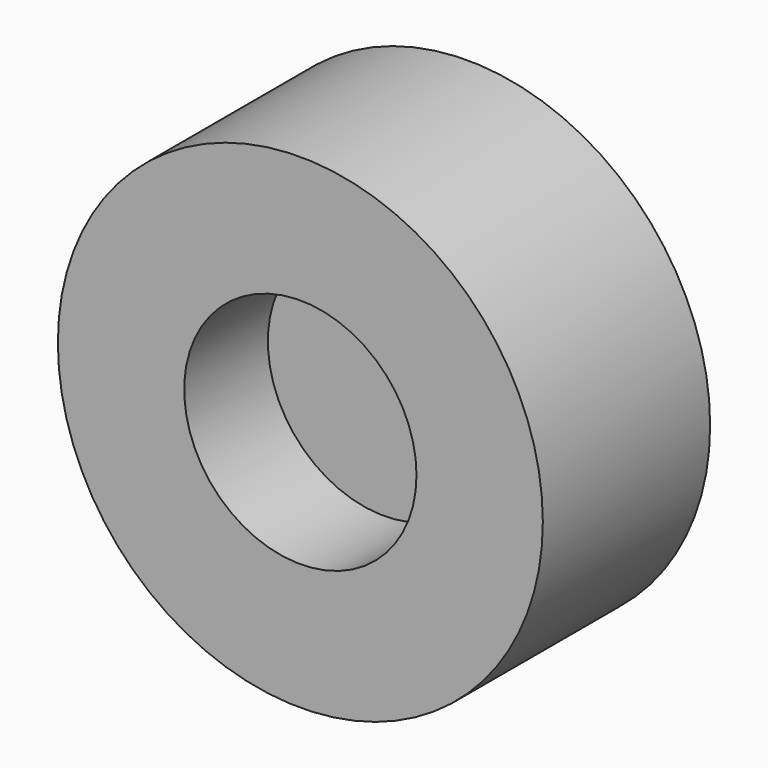
from build123d import *

# Parameters (mm, degrees)
F0_R     = 27.7693772329
F1_DEPTH = 25
F0_R_2   = 57.9777716045
F2_DEPTH = 50


# Not quite as in the source:
# - a feature of the source that left no trace in its solid (it failed there, or was rolled back) is left out


with BuildPart() as f1:
    # F0 (on Front) → F1 (new body)
    with BuildSketch(Plane.XZ):
        Circle(F0_R)
    extrude(amount=F1_DEPTH)

    # F0 (on Front) → F2 (join)
    with BuildSketch(Plane.XZ):
        Circle(F0_R_2)
        Circle(F0_R, mode=Mode.SUBTRACT)
    extrude(amount=F2_DEPTH)


solid = f1.part
